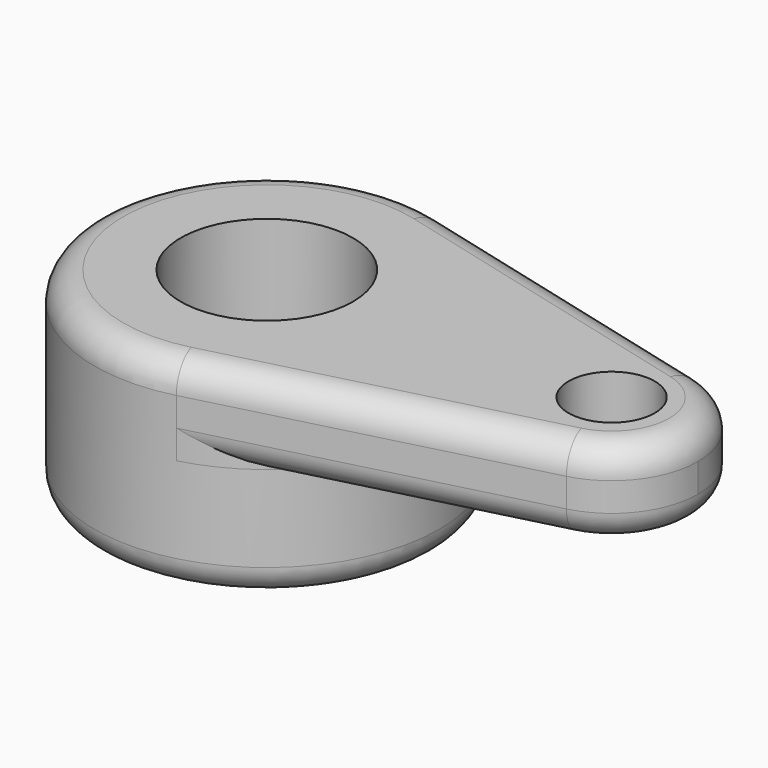
from build123d import *
from build123d import SkipClean  # not in build123d's __all__

# Parameters (mm, degrees)
F0_R         = 15
F0_R_2       = 7.5
F1_DEPTH     = 15
F2_DEPTH     = 20
F3_R         = 5
F4_T1_DEPTH  = 58.0947501931
F4_T3_DEPTH  = 58.0947501931
F4_T8_DEPTH  = 79.3447501931
F4_S9_R      = 30
F4_T10_DEPTH = 43
F4_T12_ANGLE = 151.0449756281
F4_T14_ANGLE = 151.0449756281
F4_T18_DEPTH = 79.3447501931
F4_S19_R     = 30
F4_T20_DEPTH = 43
F4_T22_ANGLE = 208.9550243719


# Not quite as in the source:
# - a fillet or chamfer that OpenCascade refuses, or shapes differently, is made with other operations: its cross-section is extruded or revolved along the edge and cut away or added


with BuildPart() as f1:
    # F0 (on Top) → F1 (new body)
    with BuildSketch(Plane.XY):
        with BuildLine():
            ThreePointArc((7.5, -29.0473750966), (23.7170824513, -18.3711730709), (30, 0))
            ThreePointArc((30, 0), (23.7170824513, 18.3711730709), (7.5, 29.0473750966))
            ThreePointArc((7.5, 29.0473750966), (-30, 0), (7.5, -29.0473750966))
        make_face()
        Circle(F0_R, mode=Mode.SUBTRACT)
        with BuildLine():
            ThreePointArc((7.5, 29.0473750966), (23.7170824513, 18.3711730709), (30, 0))
            ThreePointArc((30, 0), (23.7170824513, -18.3711730709), (7.5, -29.0473750966))
            Line((7.5, -29.0473750966), (63.75, -14.5236875483))
            ThreePointArc((63.75, -14.5236875483), (45, 0), (63.75, 14.5236875483))
            Line((63.75, 14.5236875483), (7.5, 29.0473750966))
        make_face()
        with BuildLine():
            ThreePointArc((75, 0), (71.8585412256, 9.1855865354), (63.75, 14.5236875483))
            ThreePointArc((63.75, 14.5236875483), (45, 0), (63.75, -14.5236875483))
            ThreePointArc((63.75, -14.5236875483), (71.8585412256, -9.1855865354), (75, 0))
        make_face()
        with Locations((60, 0)):
            Circle(F0_R_2, mode=Mode.SUBTRACT)
    extrude(amount=F1_DEPTH)

    # F0 (on Top) → F2 (join)
    with BuildSketch(Plane.XY):
        with BuildLine():
            ThreePointArc((7.5, -29.0473750966), (23.7170824513, -18.3711730709), (30, 0))
            ThreePointArc((30, 0), (23.7170824513, 18.3711730709), (7.5, 29.0473750966))
            ThreePointArc((7.5, 29.0473750966), (-30, 0), (7.5, -29.0473750966))
        make_face()
        Circle(F0_R, mode=Mode.SUBTRACT)
    with SkipClean():  # cleaning this boolean's faces spoils the solid; the shape is the same uncleaned
        extrude(amount=-F2_DEPTH)

    # F3
    f3_edges = [f1.edges().sort_by_distance(p)[0] for p in [
        (-7.5, 29.047375, -20),
        (-15, 0, -20),
    ]]
    fillet(f3_edges, radius=F3_R)

    # F4: fillet of radius 5 on 11 edges, made by hand

    # F4_s2 → F4_t1 (cut)
    with BuildSketch(Plane(origin=(0, 0, 0), x_dir=(0, 0, 1), z_dir=(0.9682458366, 0.25, 0))):
        with BuildLine():
            ThreePointArc((10, 30), (13.5355339059, 28.5355339059), (15, 25))
            Line((15, 25), (15, 30))
            Line((15, 30), (10, 30))
        make_face()
    extrude(amount=F4_T1_DEPTH, mode=Mode.SUBTRACT)

    # F4_s4 → F4_t3 (cut)
    with BuildSketch(Plane(origin=(56.25, -14.5236875483, 0), x_dir=(0, 0, 1), z_dir=(-0.9682458366, 0.25, 0))):
        with BuildLine():
            ThreePointArc((10, 30), (13.5355339059, 28.5355339059), (15, 25))
            Line((15, 25), (15, 30))
            Line((15, 30), (10, 30))
        make_face()
    extrude(amount=F4_T3_DEPTH, mode=Mode.SUBTRACT)


with BuildPart() as f4_tool6:
    # F4_s7 → F4_t8 (new body)
    with BuildSketch(Plane(origin=(-20.5752240267, -5.3125, 0), x_dir=(0, 0, 1), z_dir=(0.9682458366, 0.25, 0))):
        with BuildLine():
            ThreePointArc((0, 25), (1.4644660941, 28.5355339059), (5, 30))
            Line((5, 30), (0, 30))
            Line((0, 30), (0, 25))
        make_face()
    extrude(amount=F4_T8_DEPTH)

    # F4_s9 → F4_t10 (cut, symmetric)
    with BuildSketch(Plane.XY.offset(2.5)):
        Circle(F4_S9_R)
    extrude(amount=F4_T10_DEPTH, both=True, mode=Mode.SUBTRACT)


with BuildPart() as f1_1:
    add(f1.part, clean=False)

    # F4_t5: cut F4_tool6
    add(f4_tool6.part, mode=Mode.SUBTRACT)

    # F4_s11 → F4_t12 (revolve, cut)
    with BuildSketch(Plane(origin=(56.25, 14.5236875483, 0), x_dir=(0, 0, 1), z_dir=(-0.9682458366, -0.25, 0))):
        with BuildLine():
            ThreePointArc((0, -25), (1.4644660941, -28.5355339059), (5, -30))
            Line((5, -30), (0, -30))
            Line((0, -30), (0, -25))
        make_face()
    revolve(axis=Axis((60, 0, 0), (0, 0, 1)), revolution_arc=F4_T12_ANGLE, mode=Mode.SUBTRACT)

    # F4_s13 → F4_t14 (revolve, cut)
    with BuildSketch(Plane(origin=(56.25, 14.5236875483, 0), x_dir=(0, 0, 1), z_dir=(-0.9682458366, -0.25, 0))):
        with BuildLine():
            ThreePointArc((15, -25), (13.5355339059, -28.5355339059), (10, -30))
            Line((10, -30), (15, -30))
            Line((15, -30), (15, -25))
        make_face()
    revolve(axis=Axis((60, 0, 15), (0, 0, 1)), revolution_arc=F4_T14_ANGLE, mode=Mode.SUBTRACT)


with BuildPart() as f4_tool16:
    # F4_s17 → F4_t18 (new body)
    with BuildSketch(Plane(origin=(56.25, -14.5236875483, 0), x_dir=(0, 0, 1), z_dir=(-0.9682458366, 0.25, 0))):
        with BuildLine():
            ThreePointArc((0, 25), (1.4644660941, 28.5355339059), (5, 30))
            Line((5, 30), (0, 30))
            Line((0, 30), (0, 25))
        make_face()
    extrude(amount=F4_T18_DEPTH)

    # F4_s19 → F4_t20 (cut, symmetric)
    with BuildSketch(Plane.XY.offset(2.5)):
        Circle(F4_S19_R)
    extrude(amount=F4_T20_DEPTH, both=True, mode=Mode.SUBTRACT)


with BuildPart() as f1_2:
    add(f1_1.part, clean=False)

    # F4_t15: cut F4_tool16
    add(f4_tool16.part, mode=Mode.SUBTRACT)

    # F4_s21 → F4_t22 (revolve, cut)
    with BuildSketch(Plane(origin=(0, 0, 0), x_dir=(0, 0, 1), z_dir=(0.9682458366, -0.25, 0))):
        with BuildLine():
            ThreePointArc((10, -30), (13.5355339059, -28.5355339059), (15, -25))
            Line((15, -25), (15, -30))
            Line((15, -30), (10, -30))
        make_face()
    revolve(axis=Axis((0, 0, 15), (0, 0, 1)), revolution_arc=F4_T22_ANGLE, mode=Mode.SUBTRACT)


solid = f1_2.part
